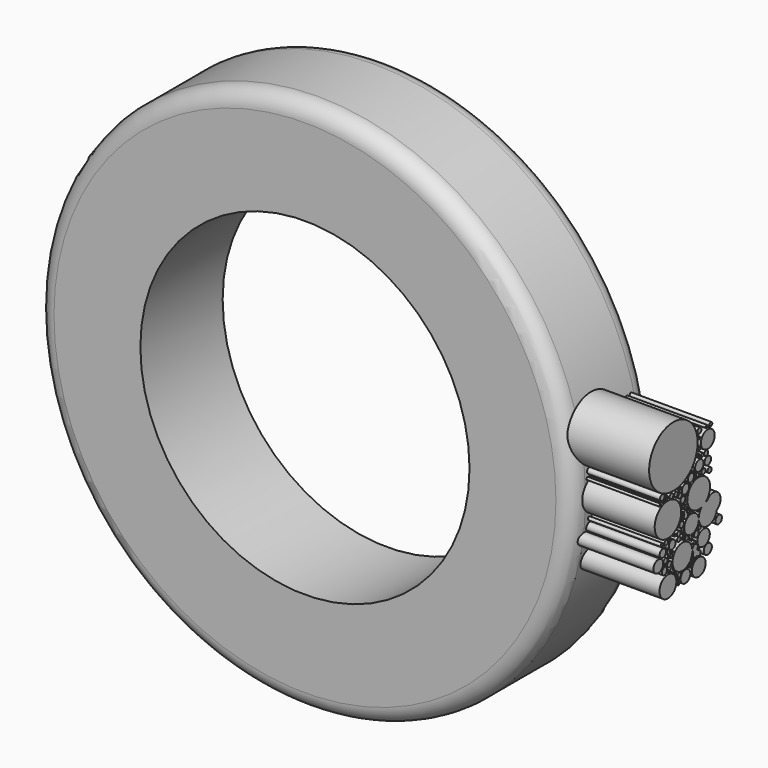
from build123d import *

# Parameters (mm, degrees)
F0_R     = 8.255
F0_R_2   = 5.08
F1_DEPTH = 3.175
F2_R     = 0.508
F4_R     = 0.9356356217
F4_R_2   = 0.3820901319
F4_R_3   = 0.2656205701
F4_R_4   = 0.511131003
F4_R_5   = 0.1863719663
F4_R_6   = 0.2398513211
F4_R_7   = 0.2656206773
F4_R_8   = 0.3244815376
F4_R_9   = 0.1630751067
F4_R_10  = 0.1254552774
F4_R_11  = 0.1562771435
F4_R_12  = 0.1254556989
F4_R_13  = 0.1317847577
F4_R_14  = 0.1878220161
F4_R_15  = 0.1417066426
F4_R_16  = 0.0789509078
F4_R_17  = 0.0419037989
F4_R_18  = 0.056285973
F4_R_19  = 0.0371865842
F4_R_20  = 0.0482972583
F4_R_21  = 0.053695609
F4_R_22  = 0.076604249
F4_R_23  = 0.1216110337
F4_R_24  = 0.0781386238
F4_R_25  = 0.0798494983
F4_R_26  = 0.0696247728
F4_R_27  = 0.0356179173
F4_R_28  = 0.0962200696
F4_R_29  = 0.0492190148
F4_R_30  = 0.0250427319
F4_R_31  = 0.0554438036
F4_R_32  = 0.02912055
F4_R_33  = 0.0230218579
F4_R_34  = 0.0350052724
F4_R_35  = 0.0723046651
F4_R_36  = 0.0242492462
F4_R_37  = 0.0276261925
F4_R_38  = 0.0602802538
F4_R_39  = 0.0545681091
F4_R_40  = 0.0218889015
F4_R_41  = 0.0277027968
F4_R_42  = 0.0730897389
F4_R_43  = 0.0231128652
F4_R_44  = 0.0231325103
F4_R_45  = 0.0857674899
F4_R_46  = 0.0387446124
F4_R_47  = 0.032547097
F4_R_48  = 0.0231130631
F4_R_49  = 0.0134771363
F4_R_50  = 0.0363207655
F4_R_51  = 0.0733791385
F4_R_52  = 0.0514441515
F4_R_53  = 0.0376097374
F4_R_54  = 0.0189179709
F4_R_55  = 0.027942021
F4_R_56  = 0.0286074303
F4_R_57  = 0.0574112711
F4_R_58  = 0.0911350383
F4_R_59  = 0.033020624
F4_R_60  = 0.0660413643
F4_R_61  = 0.0405249306
F4_R_62  = 0.0315615893
F4_R_63  = 0.0689334341
F4_R_64  = 0.0346130197
F4_R_65  = 0.0223173229
F4_R_66  = 0.1230607229
F4_R_67  = 0.0499032736
F4_R_68  = 0.0453823468
F4_R_69  = 0.0640756347
F4_R_70  = 0.0352297248
F4_R_71  = 0.0240423491
F4_R_72  = 0.021037474
F4_R_73  = 0.0147608807
F4_R_74  = 0.0222181221
F4_R_75  = 0.0181722107
F4_R_76  = 0.0350570772
F4_R_77  = 0.0116694456
F4_R_78  = 0.0147607643
F4_R_79  = 0.0430836619
F4_R_80  = 0.0315407567
F4_R_81  = 0.0665444807
F4_R_82  = 0.0203097997
F4_R_83  = 0.0317002451
F4_R_84  = 0.0812096684
F4_R_85  = 0.0303441643
F4_R_86  = 0.0515718118
F4_R_87  = 0.0771016654
F5_DEPTH = 2.54


# Not quite as in the source:
# - a length typed as a fraction of an inch, garbled in the dataset ("3 / 203.2 mm" for 3/8 in), is restored


with BuildPart() as f1:
    # F0 (on Front) → F1 (new body)
    with BuildSketch(Plane.XZ):
        Circle(F0_R)
        Circle(F0_R_2, mode=Mode.SUBTRACT)
    extrude(amount=F1_DEPTH)

    # F2
    f2_edges = [f1.edges().sort_by_distance(p)[0] for p in [
        (-8.255, -3.175, 0),
        (8.255, -1.5875, 0),
        (-8.255, 0, 0),
    ]]
    fillet(f2_edges, radius=F2_R)


with BuildPart() as f5:
    # F4 (on offset) → F5 (new body)
    with BuildSketch(Plane.YZ.offset(7.9375)):
        with Locations((-2.0558135584, 1.6283293953)):
            Circle(F4_R)
        with Locations((-1.7063668929, -1.2371331686)):
            Circle(F4_R_2)
        with BuildLine():
            ThreePointArc((-0.7982496533, -0.1066172805), (-0.6812888678, 0.0442457592), (-0.639662797, 0.2305432427))
            ThreePointArc((-0.639662797, 0.2305432427), (-1.4241092785, 0.4976547183), (-0.9656783406, -0.1926683205))
            ThreePointArc((-0.9656783406, -0.1926683205), (-0.8878596892, -0.1381716083), (-0.7982496533, -0.1066172805))
        make_face()
        with BuildLine():
            ThreePointArc((-1.0763937688, -0.491647108), (-1.0765516753, -0.4822359999), (-1.0770252172, -0.4728354867))
            ThreePointArc((-1.0770252172, -0.4728354867), (-1.5404246779, -0.2794653402), (-1.4158936902, -0.7659045521))
            ThreePointArc((-1.4158936902, -0.7659045521), (-1.3824312722, -0.759312025), (-1.3508166828, -0.772107046))
            ThreePointArc((-1.3508166828, -0.772107046), (-1.1564117557, -0.6878394324), (-1.0763937688, -0.491647108))
        make_face()
        with BuildLine():
            ThreePointArc((-0.7982496533, -0.1066172805), (-0.8878596892, -0.1381716083), (-0.9656783406, -0.1926683205))
            ThreePointArc((-0.9656783406, -0.1926683205), (-0.8772831024, -0.1587503724), (-0.7982496533, -0.1066172805))
        make_face()
        with BuildLine():
            ThreePointArc((-0.7982496533, -0.1066172805), (-0.8772831024, -0.1587503724), (-0.9656783406, -0.1926683205))
            ThreePointArc((-0.9656783406, -0.1926683205), (-1.0530743962, -0.3201443793), (-1.0770252172, -0.4728354867))
            ThreePointArc((-1.0770252172, -0.4728354867), (-0.7454673724, -0.7988281197), (-0.3829150167, -0.5076965503))
            ThreePointArc((-0.3829150167, -0.5076965503), (-0.7279162528, -0.4493720263), (-0.7533447016, -0.1004006851))
            ThreePointArc((-0.7533447016, -0.1004006851), (-0.7758979625, -0.1027809726), (-0.7982496533, -0.1066172805))
        make_face()
        with BuildLine():
            ThreePointArc((-0.3780196924, -0.4493720263), (-0.4896618969, -0.1931251436), (-0.7533447016, -0.1004006851))
            ThreePointArc((-0.7533447016, -0.1004006851), (-0.7279162528, -0.4493720263), (-0.3829150167, -0.5076965503))
            ThreePointArc((-0.3829150167, -0.5076965503), (-0.3792456713, -0.4786368273), (-0.3780196924, -0.4493720263))
        make_face()
        with BuildLine():
            ThreePointArc((-0.2348346226, -0.2586820628), (-0.4355023731, 0.0123832875), (-0.7533447016, -0.1004006851))
            ThreePointArc((-0.7533447016, -0.1004006851), (-0.4896618969, -0.1931251436), (-0.3780196924, -0.4493720263))
            ThreePointArc((-0.3780196924, -0.4493720263), (-0.3792456713, -0.4786368273), (-0.3829150167, -0.5076965503))
            ThreePointArc((-0.3829150167, -0.5076965503), (-0.2746516908, -0.4035406302), (-0.2348346226, -0.2586820628))
        make_face()
        with BuildLine():
            ThreePointArc((-1.3508166828, -0.772107046), (-1.3824312722, -0.759312025), (-1.4158936902, -0.7659045521))
            ThreePointArc((-1.4158936902, -0.7659045521), (-1.3835364772, -0.7709079139), (-1.3508166828, -0.772107046))
        make_face()
        with BuildLine():
            ThreePointArc((-1.3508166828, -0.772107046), (-1.3835364772, -0.7709079139), (-1.4158936902, -0.7659045521))
            ThreePointArc((-1.4158936902, -0.7659045521), (-1.4189777809, -0.8698931058), (-1.3283717716, -0.8187689236))
            ThreePointArc((-1.3283717716, -0.8187689236), (-1.3342747014, -0.7928792304), (-1.3508166828, -0.772107046))
        make_face()
        with Locations((-0.7279162528, 1.5584401553)):
            Circle(F4_R_3)
        with Locations((-2.2654815111, 0)):
            Circle(F4_R_4)
        with Locations((-2.6382245123, -1.1206504423)):
            Circle(F4_R_5)
        with Locations((-0.8909913595, -1.0507612024)):
            Circle(F4_R_6)
        with Locations((-1.0773630347, -1.7729505198)):
            Circle(F4_R_7)
        with Locations((-2.2654815111, -1.8195440061)):
            Circle(F4_R_8)
        with Locations((-1.0540664662, 0.9760293178)):
            Circle(F4_R_9)
        with Locations((-0.7279162528, 0.9760293178)):
            Circle(F4_R_10)
        with Locations((-0.7279162528, -1.4235042036)):
            Circle(F4_R_11)
        with Locations((-0.3085803473, -0.7944998797)):
            Circle(F4_R_12)
        with Locations((-2.1024062298, -0.7479073829)):
            Circle(F4_R_13)
        with Locations((-1.5898846323, -1.8195440061)):
            Circle(F4_R_14)
        with Locations((-1.5898846323, 0.5566932959)):
            Circle(F4_R_15)
        with Locations((-1.0540664662, 1.9191203173)):
            Circle(F4_R_16)
        with Locations((-0.773440639, 1.9191203173)):
            Circle(F4_R_17)
        with Locations((-0.6103655323, 1.9191203173)):
            Circle(F4_R_18)
        with Locations((-1.0540664662, 1.7230617814)):
            Circle(F4_R_19)
        with Locations((-1.0540664662, 1.4376804465)):
            Circle(F4_R_20)
        with Locations((-0.9423398296, 1.216364326)):
            Circle(F4_R_21)
        with Locations((-0.7909130072, 1.2047159253)):
            Circle(F4_R_22)
        with Locations((-1.3791481033, 0.7737317937)):
            Circle(F4_R_23)
        with Locations((-0.6569584366, 0.6921943859)):
            Circle(F4_R_24)
        with Locations((-0.8909913595, 0.7504355162)):
            Circle(F4_R_25)
        with Locations((-1.9557350315, 0.5566932959)):
            Circle(F4_R_26)
        with Locations((-1.0773630347, 1.2629571138)):
            Circle(F4_R_27)
        with Locations((-1.6934229061, 0.3039045841)):
            Circle(F4_R_28)
        with Locations((-1.6640380491, 0.093313145)):
            Circle(F4_R_29)
        with BuildLine():
            ThreePointArc((-1.5364069236, -0.1091672266), (-1.5301660872, -0.094186667), (-1.5280369438, -0.0780984119))
            ThreePointArc((-1.5280369438, -0.0780984119), (-1.6151773372, -0.0216589253), (-1.6310453416, -0.1242604372))
            ThreePointArc((-1.6310453416, -0.1242604372), (-1.5861129065, -0.101748129), (-1.5364069236, -0.1091672266))
        make_face()
        with BuildLine():
            ThreePointArc((-1.5364069236, -0.1091672266), (-1.5861129065, -0.101748129), (-1.6310453416, -0.1242604372))
            ThreePointArc((-1.6310453416, -0.1242604372), (-1.5801440794, -0.1391742516), (-1.5364069236, -0.1091672266))
        make_face()
        with BuildLine():
            ThreePointArc((-1.5364069236, -0.1091672266), (-1.5801440794, -0.1391742516), (-1.6310453416, -0.1242604372))
            ThreePointArc((-1.6310453416, -0.1242604372), (-1.6054399021, -0.2607914789), (-1.4896581574, -0.184038945))
            ThreePointArc((-1.4896581574, -0.184038945), (-1.5023050403, -0.1399049973), (-1.5364069236, -0.1091672266))
        make_face()
        with Locations((-1.5171138803, 0)):
            Circle(F4_R_30)
        with Locations((-1.5729889274, 0.1725616166)):
            Circle(F4_R_31)
        with Locations((-1.5709298896, 0.3640611249)):
            Circle(F4_R_32)
        with Locations((-1.7294831341, 0.1581477554)):
            Circle(F4_R_33)
        with Locations((-1.8468537601, 0.5905658472)):
            Circle(F4_R_34)
        with Locations((-1.8015528331, 0.4546630371)):
            Circle(F4_R_35)
        with Locations((-1.5898846323, 0.7532374584)):
            Circle(F4_R_36)
        with Locations((-1.4000217197, 0.5905658472)):
            Circle(F4_R_37)
        with Locations((-1.126156887, 0.7532374584)):
            Circle(F4_R_38)
        with Locations((-1.3032424031, 0.9760293178)):
            Circle(F4_R_39)
        with Locations((-1.2249953579, 0.8520758711)):
            Circle(F4_R_40)
        with Locations((-1.2373501668, 0.6914634141)):
            Circle(F4_R_41)
        with Locations((-2.1276406478, 0.583070796)):
            Circle(F4_R_42)
        with Locations((-2.2801866289, 0.6223627715)):
            Circle(F4_R_43)
        with Locations((-2.3241012823, 0.5566932959)):
            Circle(F4_R_44)
        with Locations((-2.48358096, 0.6847679033)):
            Circle(F4_R_45)
        with Locations((-2.5621650275, 0.5067978636)):
            Circle(F4_R_46)
        with Locations((-2.4512226228, 0.5566932959)):
            Circle(F4_R_47)
        with Locations((-2.3680159356, 0.6269854493)):
            Circle(F4_R_48)
        with Locations((-2.3495254572, 0.7055696333)):
            Circle(F4_R_49)
        with Locations((-1.7808944685, 0.6539656897)):
            Circle(F4_R_50)
        with BuildLine():
            ThreePointArc((-1.714935524, -0.2677784606), (-1.8114776347, -0.4058317685), (-1.6515779488, -0.3528111556))
            ThreePointArc((-1.6515779488, -0.3528111556), (-1.66915888, -0.2997905427), (-1.714935524, -0.2677784606))
        make_face()
        with BuildLine():
            ThreePointArc((-1.6764101979, -0.2390733716), (-1.7242654362, -0.2150515957), (-1.714935524, -0.2677784606))
            ThreePointArc((-1.714935524, -0.2677784606), (-1.6884683496, -0.2630951476), (-1.6764101979, -0.2390733716))
        make_face()
        with Locations((-1.8503870815, -0.5546038738)):
            Circle(F4_R_51)
        with Locations((-1.7063668929, -0.5032384652)):
            Circle(F4_R_52)
        with Locations((-1.7063668929, -0.0519564528)):
            Circle(F4_R_53)
        with Locations((-1.7063668929, -0.1546872809)):
            Circle(F4_R_54)
        with Locations((-1.4284566278, -0.1473493321)):
            Circle(F4_R_55)
        with Locations((-1.0773630347, -0.2390733716)):
            Circle(F4_R_56)
        with Locations((-1.0540664662, -0.712369103)):
            Circle(F4_R_57)
        with Locations((-1.1679605814, -0.8371138247)):
            Circle(F4_R_58)
        with Locations((-1.3477395987, -0.9178309119)):
            Circle(F4_R_59)
        with Locations((-1.5385254519, -0.7967551937)):
            Circle(F4_R_60)
        with Locations((-1.6742770094, -0.7087002741)):
            Circle(F4_R_61)
        with Locations((-1.6816149, -0.6023003371)):
            Circle(F4_R_62)
        with Locations((-1.8467181362, -0.7050312706)):
            Circle(F4_R_63)
        with Locations((-1.9861385226, -0.5435969797)):
            Circle(F4_R_64)
        with Locations((-2.1879314445, -0.6023003371)):
            Circle(F4_R_65)
        with Locations((-2.3310207762, -0.6023003371)):
            Circle(F4_R_51)
        with Locations((-2.463103272, -0.8371138247)):
            Circle(F4_R_66)
        with Locations((-2.4961240124, -0.6023003371)):
            Circle(F4_R_67)
        with Locations((-2.2429658566, -1.0315686231)):
            Circle(F4_R_68)
        with Locations((-2.2466348018, -0.895817182)):
            Circle(F4_R_69)
        with Locations((-2.1024062298, -0.9435136453)):
            Circle(F4_R_70)
        with BuildLine():
            ThreePointArc((-1.2165080051, -1.0969773462), (-1.1922372732, -1.0793129032), (-1.1829689751, -1.0507612024))
            ThreePointArc((-1.1829689751, -1.0507612024), (-1.2638558077, -1.0144092927), (-1.2373366784, -1.0990312568))
            ThreePointArc((-1.2373366784, -1.0990312568), (-1.2269744057, -1.0974763217), (-1.2165080051, -1.0969773462))
        make_face()
        with BuildLine():
            ThreePointArc((-1.2165080051, -1.0969773462), (-1.2269744057, -1.0974763217), (-1.2373366784, -1.0990312568))
            ThreePointArc((-1.2373366784, -1.0990312568), (-1.2268104927, -1.099138561), (-1.2165080051, -1.0969773462))
        make_face()
        with BuildLine():
            ThreePointArc((-1.2165080051, -1.0969773462), (-1.2268104927, -1.099138561), (-1.2373366784, -1.0990312568))
            ThreePointArc((-1.2373366784, -1.0990312568), (-1.3177546201, -1.1776667179), (-1.2789148994, -1.2832226613))
            ThreePointArc((-1.2789148994, -1.2832226613), (-1.2115953042, -1.2486352161), (-1.1384266614, -1.2679890008))
            ThreePointArc((-1.1384266614, -1.2679890008), (-1.1198185449, -1.2364733296), (-1.1133459176, -1.20045105))
            ThreePointArc((-1.1133459176, -1.20045105), (-1.1435425453, -1.1273941823), (-1.2165080051, -1.0969773462))
        make_face()
        with BuildLine():
            ThreePointArc((-1.1384266614, -1.2679890008), (-1.2115953042, -1.2486352161), (-1.2789148994, -1.2832226613))
            ThreePointArc((-1.2789148994, -1.2832226613), (-1.2056653897, -1.3033222188), (-1.1384266614, -1.2679890008))
        make_face()
        with BuildLine():
            ThreePointArc((-1.1384266614, -1.2679890008), (-1.2056653897, -1.3033222188), (-1.2789148994, -1.2832226613))
            ThreePointArc((-1.2789148994, -1.2832226613), (-1.2962252557, -1.3975028708), (-1.1984570464, -1.459155056))
            ThreePointArc((-1.1984570464, -1.459155056), (-1.1860071032, -1.4544645144), (-1.1727459199, -1.4555337596))
            ThreePointArc((-1.1727459199, -1.4555337596), (-1.1593167597, -1.4509264934), (-1.1466272027, -1.4445590456))
            ThreePointArc((-1.1466272027, -1.4445590456), (-1.1613481271, -1.3665501889), (-1.1027660092, -1.3129757286))
            ThreePointArc((-1.1027660092, -1.3129757286), (-1.1174799499, -1.2880120286), (-1.1384266614, -1.2679890008))
        make_face()
        with BuildLine():
            ThreePointArc((-1.1727459199, -1.4555337596), (-1.1860071032, -1.4544645144), (-1.1984570464, -1.459155056))
            ThreePointArc((-1.1984570464, -1.459155056), (-1.1854897322, -1.4581378374), (-1.1727459199, -1.4555337596))
        make_face()
        with BuildLine():
            ThreePointArc((-1.1727459199, -1.4555337596), (-1.1854897322, -1.4581378374), (-1.1984570464, -1.459155056))
            ThreePointArc((-1.1984570464, -1.459155056), (-1.1962198634, -1.5113744129), (-1.1513326654, -1.4845974511))
            ThreePointArc((-1.1513326654, -1.4845974511), (-1.1572640402, -1.4665473428), (-1.1727459199, -1.4555337596))
        make_face()
        with BuildLine():
            ThreePointArc((-1.0946392897, -1.3535948237), (-1.0966909039, -1.3328827834), (-1.1027660092, -1.3129757286))
            ThreePointArc((-1.1027660092, -1.3129757286), (-1.1613481271, -1.3665501889), (-1.1466272027, -1.4445590456))
            ThreePointArc((-1.1466272027, -1.4445590456), (-1.1085531289, -1.4059809688), (-1.0946392897, -1.3535948237))
        make_face()
        with BuildLine():
            ThreePointArc((-1.0024112022, -1.3923421502), (-1.0333789238, -1.3283692728), (-1.1027660092, -1.3129757286))
            ThreePointArc((-1.1027660092, -1.3129757286), (-1.0966909039, -1.3328827834), (-1.0946392897, -1.3535948237))
            ThreePointArc((-1.0946392897, -1.3535948237), (-1.1085531289, -1.4059809688), (-1.1466272027, -1.4445590456))
            ThreePointArc((-1.1466272027, -1.4445590456), (-1.0562052602, -1.4690312286), (-1.0024112022, -1.3923421502))
        make_face()
        with BuildLine():
            ThreePointArc((-1.3229980364, -1.5329247116), (-1.2920375712, -1.5260574638), (-1.2782195311, -1.4975132653))
            ThreePointArc((-1.2782195311, -1.4975132653), (-1.3304241466, -1.4647374668), (-1.3372587294, -1.5259980849))
            ThreePointArc((-1.3372587294, -1.5259980849), (-1.3297543984, -1.5286914307), (-1.3229980364, -1.5329247116))
        make_face()
        with BuildLine():
            ThreePointArc((-1.3229980364, -1.5329247116), (-1.3297543984, -1.5286914307), (-1.3372587294, -1.5259980849))
            ThreePointArc((-1.3372587294, -1.5259980849), (-1.3305101663, -1.5302474224), (-1.3229980364, -1.5329247116))
        make_face()
        with BuildLine():
            ThreePointArc((-1.3229980364, -1.5329247116), (-1.3305101663, -1.5302474224), (-1.3372587294, -1.5259980849))
            ThreePointArc((-1.3372587294, -1.5259980849), (-1.3751540199, -1.5850597958), (-1.3088455097, -1.5620919876))
            ThreePointArc((-1.3088455097, -1.5620919876), (-1.3125704802, -1.5458822374), (-1.3229980364, -1.5329247116))
        make_face()
        with Locations((-1.3164558914, -1.4218639117)):
            Circle(F4_R_71)
        with Locations((-1.0692115175, -1.2613395229)):
            Circle(F4_R_72)
        with Locations((-1.246341737, -1.4975132653)):
            Circle(F4_R_73)
        with Locations((-1.3939503115, -1.4956680825)):
            Circle(F4_R_74)
        with Locations((-1.4253171394, -1.5473311068)):
            Circle(F4_R_75)
        with Locations((-1.3662737329, -1.643276657)):
            Circle(F4_R_76)
        with Locations((-1.4345427044, -1.6156000784)):
            Circle(F4_R_73)
        with Locations((-1.4769801637, -1.6082195798)):
            Circle(F4_R_77)
        with Locations((-1.4659095323, -1.5657822369)):
            Circle(F4_R_78)
        with Locations((-1.862622099, -1.9057360478)):
            Circle(F4_R_79)
        with Locations((-1.8800375983, -1.7977599055)):
            Circle(F4_R_80)
        with Locations((-1.8277911004, -1.6828178195)):
            Circle(F4_R_81)
        with Locations((-1.9288009498, -1.6479868209)):
            Circle(F4_R_82)
        with Locations((-1.9775643013, -1.5620919876)):
            Circle(F4_R_83)
        with BuildLine():
            ThreePointArc((-2.0956454203, -1.4734366016), (-2.0829946113, -1.5247565169), (-2.0394951124, -1.4947303571))
            ThreePointArc((-2.0394951124, -1.4947303571), (-2.0529408363, -1.4686004751), (-2.0820184606, -1.4643519473))
            ThreePointArc((-2.0820184606, -1.4643519473), (-2.0885065233, -1.4693823994), (-2.0956454203, -1.4734366016))
        make_face()
        with BuildLine():
            ThreePointArc((-2.0956454203, -1.4734366016), (-2.0885065233, -1.4693823994), (-2.0820184606, -1.4643519473))
            ThreePointArc((-2.0820184606, -1.4643519473), (-2.0894208238, -1.4680109508), (-2.0956454203, -1.4734366016))
        make_face()
        with BuildLine():
            ThreePointArc((-2.0956454203, -1.4734366016), (-2.0894208238, -1.4680109508), (-2.0820184606, -1.4643519473))
            ThreePointArc((-2.0820184606, -1.4643519473), (-2.0679161163, -1.4450027511), (-2.0629263928, -1.4215854462))
            ThreePointArc((-2.0629263928, -1.4215854462), (-2.1689524578, -1.3909297898), (-2.0956454203, -1.4734366016))
        make_face()
        with Locations((-2.2144149989, -1.2371331686)):
            Circle(F4_R_84)
        with BuildLine():
            ThreePointArc((-2.3947777976, -1.2504892226), (-2.4771159264, -1.421071004), (-2.300774419, -1.351923449))
            ThreePointArc((-2.300774419, -1.351923449), (-2.3107992336, -1.3078881191), (-2.3388978795, -1.2725317436))
            ThreePointArc((-2.3388978795, -1.2725317436), (-2.3718484008, -1.2742127422), (-2.3947777976, -1.2504892226))
        make_face()
        with BuildLine():
            ThreePointArc((-2.3947777976, -1.2504892226), (-2.3718484008, -1.2742127422), (-2.3388978795, -1.2725317436))
            ThreePointArc((-2.3388978795, -1.2725317436), (-2.3651737339, -1.2572918173), (-2.3947777976, -1.2504892226))
        make_face()
        with BuildLine():
            ThreePointArc((-2.3947777976, -1.2504892226), (-2.3651737339, -1.2572918173), (-2.3388978795, -1.2725317436))
            ThreePointArc((-2.3388978795, -1.2725317436), (-2.3231688086, -1.2578506875), (-2.3173617879, -1.2371331686))
            ThreePointArc((-2.3173617879, -1.2371331686), (-2.3639985885, -1.1978533305), (-2.3947777976, -1.2504892226))
        make_face()
        with Locations((-2.2353136446, -1.4235042036)):
            Circle(F4_R_85)
        with Locations((-2.1273375023, -1.0507612024)):
            Circle(F4_R_86)
        with Locations((-2.3607050534, -1.0872080456)):
            Circle(F4_R_87)
    extrude(amount=F5_DEPTH)


solid = Compound([f1.part, f5.part])
